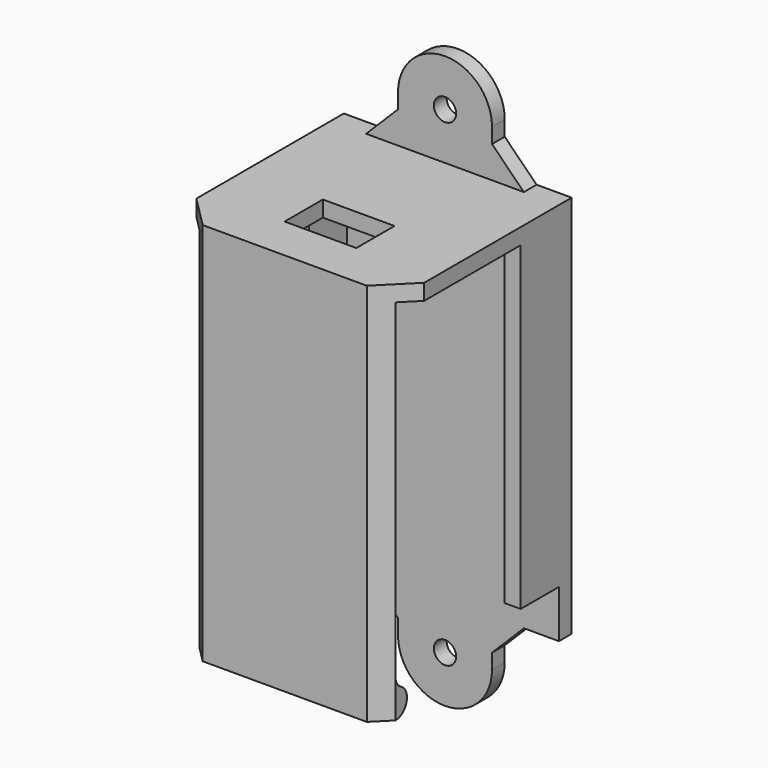
from build123d import *

# Parameters (mm, degrees)
F1_DEPTH       = 2.54
F3_DEPTH       = 36.322
F4_W           = 2.5400000004
F4_H           = 53.594
F4_W_2         = 2.5400000003
F4_H_2         = 51.054
F5_DEPTH       = 7.62
F6_R           = 2.032
F7_SIZE        = 5.08
F8_SIZE        = 5.08
F10_DEPTH      = 31.9278
F12_R          = 1.778
F13_DEPTH      = 2.54
F14_SIZE       = 5.08
F16_DEPTH      = 2.54
F16_DEPTH_BACK = 25.4


with BuildPart() as f1:
    # F0 (on Front) → F1 (new body)
    with BuildSketch(Plane.XZ):
        Polygon((18.161, 9.3117938122), (18.161, 30.607), (-18.161, 30.607), (-18.161, 9.3117938122), (-18.161, -9.3117938122), (-18.161, -30.607), (18.161, -30.607), (18.161, -9.3117938122), align=None)
    extrude(amount=F1_DEPTH)

    # F2 (on face) → F3 (join, through all)
    with BuildSketch(Plane.YZ.offset(18.161)):
        Polygon((-2.54, 28.067), (-2.54, 30.607), (-34.4678, 30.607), (-34.4678, -30.607), (-31.9278, -30.607), (-31.9278, -26.035), (-31.9278, 28.067), align=None)
        with BuildLine():
            ThreePointArc((-31.9278, -30.607), (-29.6418, -28.321), (-31.9278, -26.035))
            Line((-31.9278, -26.035), (-31.9278, -30.607))
        make_face()
    extrude(amount=-F3_DEPTH)

    # F4 (on face) → F5 (join)
    with BuildSketch(Plane.XZ.offset(2.54)):
        with Locations((-16.8910000002, 1.27)):
            Rectangle(F4_W, F4_H)
        with Locations((16.8909999998, 2.54)):
            Rectangle(F4_W_2, F4_H_2)
    extrude(amount=F5_DEPTH)

    # F6
    f6_edges = [f1.edges().sort_by_distance(p)[0] for p in [
        (0, -31.9278, -30.607),
        (0, -31.9278, -26.035),
    ]]
    fillet(f6_edges, radius=F6_R)

    # F7
    f7_edges = [f1.edges().sort_by_distance(p)[0] for p in [
        (18.161, -34.4678, 0),
    ]]
    chamfer(f7_edges, length=F7_SIZE)

    # F8
    f8_edges = [f1.edges().sort_by_distance(p)[0] for p in [
        (-18.161, -34.4678, 0),
    ]]
    chamfer(f8_edges, length=F8_SIZE)

    # F9 (on face) → F10 (cut, through all)
    with BuildSketch(Plane.XZ.offset(34.4678)):
        with BuildLine():
            ThreePointArc((-15.621, -24.511), (-15.910574375, -25.556455375), (-16.6967647059, -26.3039411765))
            ThreePointArc((-16.6967647059, -26.3039411765), (-17.8387457553, -28.8754364388), (-15.621, -30.607))
            Line((-15.621, -30.607), (-15.621, -24.511))
        make_face()
        with BuildLine():
            ThreePointArc((15.621, -30.607), (17.8387457553, -28.8754364388), (16.6967647059, -26.3039411765))
            ThreePointArc((16.6967647059, -26.3039411765), (15.910574375, -25.556455375), (15.621, -24.511))
            Line((15.621, -24.511), (15.621, -30.607))
        make_face()
    extrude(amount=-F10_DEPTH, mode=Mode.SUBTRACT)

    # F12 (on face) → F13 (join, through all)
    with BuildSketch(Plane(origin=(0, 0, 0), x_dir=(-1, 0, 0), z_dir=(0, 1, 0))):
        with BuildLine():
            Line((-7.493, 38.1), (-7.493, 30.607))
            Line((-7.493, 30.607), (7.493, 30.607))
            Line((7.493, 30.607), (7.493, 38.1))
            ThreePointArc((7.493, 38.1), (0, 45.593), (-7.493, 38.1))
        make_face()
        with Locations((0, 38.1)):
            Circle(F12_R, mode=Mode.SUBTRACT)
        with BuildLine():
            Line((-6.35, -30.607), (-7.493, -30.607))
            Line((-7.493, -30.607), (-7.493, -38.1))
            ThreePointArc((-7.493, -38.1), (0, -45.593), (7.493, -38.1))
            Line((7.493, -38.1), (7.493, -30.607))
            Line((7.493, -30.607), (6.35, -30.607))
            Line((6.35, -30.607), (0, -30.607))
            Line((0, -30.607), (-6.35, -30.607))
        make_face()
        with Locations((0, -38.1)):
            Circle(F12_R, mode=Mode.SUBTRACT)
    extrude(amount=-F13_DEPTH)

    # F14
    f14_edges = [f1.edges().sort_by_distance(p)[0] for p in [
        (-7.493, -1.27, -30.607),
        (7.493, -1.27, -30.607),
        (7.493, -1.27, 30.607),
        (-7.493, -1.27, 30.607),
    ]]
    chamfer(f14_edges, length=F14_SIZE)

    # F15 (on face) → F16 (cut, two sides)
    with BuildSketch(Plane(origin=(0, 0, 28.067), x_dir=(1, 0, 0), z_dir=(0, 0, -1))) as f16_sk:
        Polygon((5.715, 27.3558), (0, 27.3558), (-5.715, 27.3558), (-5.715, 19.7358), (5.715, 19.7358), align=None)
    extrude(amount=-F16_DEPTH, mode=Mode.SUBTRACT)
    extrude(f16_sk.sketch, amount=F16_DEPTH_BACK, mode=Mode.SUBTRACT)


solid = f1.part
